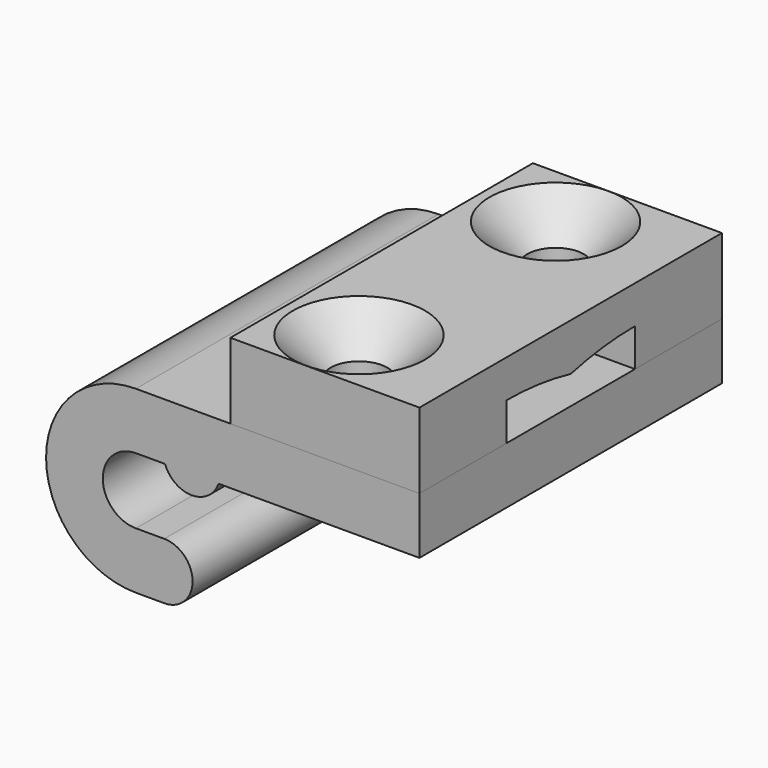
from build123d import *

# Parameters (mm, degrees)
F1_DEPTH  = 20
F2_R      = 1.5
F3_DEPTH  = 9.501
F4_W      = 10
F4_H      = 5.75
F4_R      = 1.5
F5_DEPTH  = 2
F6_W      = 10
F6_H      = 5.75
F6_R      = 1.5
F6_H_2    = 14.25
F7_DEPTH  = 2
F8_SIZE   = 1.99999
F10_DEPTH = 10


# Not quite as in the source:
# - a fillet or chamfer is up to 0.001 mm smaller than in the source, because OpenCascade refuses the exact size


with BuildPart() as f1:
    # F0 (on Front) → F1 (new body)
    with BuildSketch(Plane.XZ):
        with BuildLine():
            ThreePointArc((0, -1.75), (-1.75, 0), (0, 1.75))
            Line((0, 1.75), (1.5446865, 1.75))
            Line((1.5446865, 1.75), (4.3731136247, 1.75))
            Line((4.3731136247, 1.75), (15, 1.75))
            Line((15, 1.75), (15, 4.75))
            Line((15, 4.75), (0, 4.75))
            ThreePointArc((0, 4.75), (-4.75, 0), (0, -4.75))
            Line((0, -4.75), (1.5, -4.75))
            ThreePointArc((1.5, -4.75), (3, -3.25), (1.5, -1.75))
            Line((1.5, -1.75), (0, -1.75))
        make_face()
        with BuildLine():
            Line((4.3731136247, 1.75), (1.5446865, 1.75))
            ThreePointArc((1.5446865, 1.75), (2.9589000624, 0.75), (4.3731136247, 1.75))
        make_face()
    extrude(amount=F1_DEPTH)

    # F2 (on face) → F3 (cut, through all)
    with BuildSketch(Plane.XY.offset(4.75)):
        with Locations((9, -3.5)):
            Circle(F2_R)
        with Locations((9, -16.5)):
            Circle(F2_R)
    extrude(amount=-F3_DEPTH, mode=Mode.SUBTRACT)


with BuildPart() as f5:
    # F4 (on face) → F5 (new body)
    with BuildSketch(Plane.XY.offset(4.75)):
        with Locations((10, -2.875)):
            Rectangle(F4_W, F4_H)
        with Locations((9, -3.5)):
            Circle(F4_R, mode=Mode.SUBTRACT)
    extrude(amount=F5_DEPTH)



with BuildPart() as f5b:
    # F4 (on face) → F5, piece 2 (new body)
    with BuildSketch(Plane.XY.offset(4.75)):
        with Locations((10, -17.125)):
            Rectangle(F4_W, F4_H)
        with Locations((9, -16.5)):
            Circle(F4_R, mode=Mode.SUBTRACT)
    extrude(amount=F5_DEPTH)


with BuildPart() as f5_1:
    add(f5.part)

    add(f5b.part)  # F7 merges F5b
    # F6 (on face) → F7 (join)
    with BuildSketch(Plane.XY.offset(6.75)):
        with Locations((10, -2.875)):
            Rectangle(F6_W, F6_H)
        with Locations((9, -3.5)):
            Circle(F6_R, mode=Mode.SUBTRACT)
        with Locations((10, -12.875)):
            Rectangle(F6_W, F6_H_2)
        with Locations((9, -16.5)):
            Circle(F6_R, mode=Mode.SUBTRACT)
    extrude(amount=F7_DEPTH)

    # F8 (size 2 in the source; OpenCascade refuses exactly that, so slightly less here)
    f8_edges = [f5_1.edges().sort_by_distance(p)[0] for p in [
        (7.5, -16.5, 8.75),
        (7.5, -3.5, 8.75),
    ]]
    chamfer(f8_edges, length=F8_SIZE)

    # F9 (on face) → F10 (join, through all)
    with BuildSketch(Plane.YZ.offset(15)):
        with BuildLine():
            Line((-5.75, 6.75), (-14.25, 6.75))
            ThreePointArc((-14.25, 6.75), (-12.1103446539, 6.6245704417), (-10, 6.25))
            ThreePointArc((-10, 6.25), (-7.8896553461, 6.6245704417), (-5.75, 6.75))
        make_face()
    extrude(amount=-F10_DEPTH)


solid = Compound([f1.part, f5_1.part])
